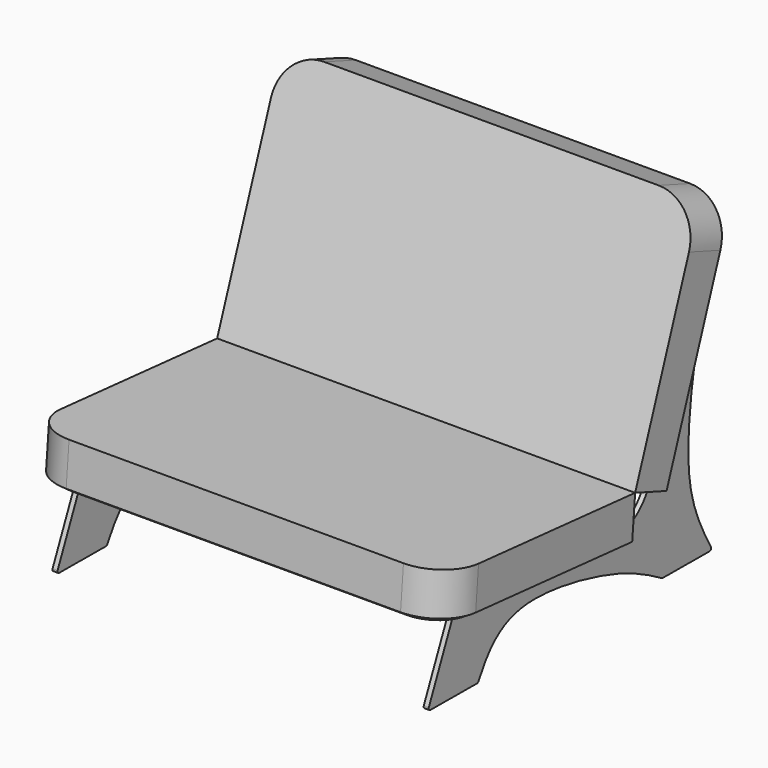
from build123d import *

# Parameters (mm, degrees)
F1_DEPTH      = 500
F1_DEPTH_BACK = 500
F2_R          = 100
F2_2_R        = 100
F4_DEPTH      = 12
F6_DEPTH      = 12
F8_START      = 438
F8_DEPTH      = 12
F10_DEPTH     = 12
F12_DEPTH     = 12
F13_R         = 5
F14_R         = 2
F15_R         = 5
F15_2_R       = 5


with BuildPart() as f1:
    # F0 (on Right) → F1 (new body, two sides)
    with BuildSketch(Plane.YZ) as f1_sk:
        Polygon((-567.8027826631, 50), (0, 0), (8.7719298246, 99.6145232742), (-559.0308528386, 149.6145232742), align=None)
    extrude(amount=F1_DEPTH)
    extrude(f1_sk.sketch, amount=-F1_DEPTH_BACK)

    # F2
    f2_edges = [f1.edges().sort_by_distance(p)[0] for p in [
        (-500, -563.416818, 99.807262),
        (500, -563.416818, 99.807262),
    ]]
    fillet(f2_edges, radius=F2_R)


with BuildPart() as f1b:
    # F0 (on Right) → F1, piece 2 (new body, two sides)
    with BuildSketch(Plane.YZ) as f1_2_sk:
        Polygon((204.0263951544, 635.1289430322), (8.7719298246, 99.6145232742), (102.7218280277, 65.3593539181), (297.9762933576, 600.8737736761), align=None)
    extrude(amount=F1_DEPTH)
    extrude(f1_2_sk.sketch, amount=-F1_DEPTH_BACK)

    # F2#2
    f2_2_edges = [f1b.edges().sort_by_distance(p)[0] for p in [
        (500, 251.001344, 618.001358),
        (-500, 251.001344, 618.001358),
    ]]
    fillet(f2_2_edges, radius=F2_2_R)


with BuildPart() as f4:
    # F3 (on face) → F4 (new body)
    with BuildSketch(Plane(origin=(0, 0, 0), x_dir=(1, 0, 0), z_dir=(0, -0.0877192982, -0.9961452327))):
        with BuildLine():
            Line((-480, 20), (480, 20))
            Line((480, 20), (480, 470))
            ThreePointArc((480, 470), (456.5685424949, 526.5685424949), (400, 550))
            Line((400, 550), (-400, 550))
            ThreePointArc((-400, 550), (-456.5685424949, 526.5685424949), (-480, 470))
            Line((-480, 470), (-480, 20))
        make_face()
    extrude(amount=F4_DEPTH)

    # F9 (on face) → F10 (cut, through all)
    with BuildSketch(Plane(origin=(0, 0, 0), x_dir=(1, 0, 0), z_dir=(0, 0.0877192982, 0.9961452327))):
        with BuildLine():
            Line((438, -51), (438, -79))
            ThreePointArc((438, -79), (437.2928932188, -80.7071067812), (439, -80))
            Line((439, -80), (449, -80))
            ThreePointArc((449, -80), (450.7071067812, -80.7071067812), (450, -79))
            Line((450, -79), (450, -51))
            ThreePointArc((450, -51), (450.7071067812, -49.2928932188), (449, -50))
            Line((449, -50), (439, -50))
            ThreePointArc((439, -50), (437.2928932188, -49.2928932188), (438, -51))
        make_face()
        with BuildLine():
            Line((438, -411), (438, -439))
            ThreePointArc((438, -439), (437.2928932188, -440.7071067812), (439, -440))
            Line((439, -440), (449, -440))
            ThreePointArc((449, -440), (450.7071067812, -440.7071067812), (450, -439))
            Line((450, -439), (450, -411))
            ThreePointArc((450, -411), (450.7071067812, -409.2928932188), (449, -410))
            Line((449, -410), (439, -410))
            ThreePointArc((439, -410), (437.2928932188, -409.2928932188), (438, -411))
        make_face()
        with BuildLine():
            ThreePointArc((-449, -410), (-450.7071067812, -409.2928932188), (-450, -411))
            Line((-450, -411), (-450, -439))
            ThreePointArc((-450, -439), (-450.7071067812, -440.7071067812), (-449, -440))
            Line((-449, -440), (-439, -440))
            ThreePointArc((-439, -440), (-437.2928932188, -440.7071067812), (-438, -439))
            Line((-438, -439), (-438, -411))
            ThreePointArc((-438, -411), (-437.2928932188, -409.2928932188), (-439, -410))
            Line((-439, -410), (-449, -410))
        make_face()
        with BuildLine():
            ThreePointArc((-450, -79), (-450.7071067812, -80.7071067812), (-449, -80))
            Line((-449, -80), (-439, -80))
            ThreePointArc((-439, -80), (-437.2928932188, -80.7071067812), (-438, -79))
            Line((-438, -79), (-438, -51))
            ThreePointArc((-438, -51), (-437.2928932188, -49.2928932188), (-439, -50))
            Line((-439, -50), (-449, -50))
            ThreePointArc((-449, -50), (-450.7071067812, -49.2928932188), (-450, -51))
            Line((-450, -51), (-450, -79))
        make_face()
    extrude(amount=-F10_DEPTH, mode=Mode.SUBTRACT)

    # F15
    f15_edges = [f4.edges().sort_by_distance(p)[0] for p in [
        (-480, -20.44922, -4.222485),
        (480, -20.44922, -4.222485),
    ]]
    fillet(f15_edges, radius=F15_R)


with BuildPart() as f6:
    # F5 (on face) → F6 (new body)
    with BuildSketch(Plane(origin=(0, 69.6338752627, -25.3892791335), x_dir=(-1, 0, 0), z_dir=(0, 0.939498982, -0.3425516936))):
        with BuildLine():
            Line((400, 646.5925826289), (-400, 646.5925826289))
            ThreePointArc((-400, 646.5925826289), (-456.5685424949, 623.1611251238), (-480, 566.5925826289))
            Line((-480, 566.5925826289), (-480, 346.5925826289))
            Line((-480, 346.5925826289), (480, 346.5925826289))
            Line((480, 346.5925826289), (480, 566.5925826289))
            ThreePointArc((480, 566.5925826289), (456.5685424949, 623.1611251238), (400, 646.5925826289))
        make_face()
    extrude(amount=F6_DEPTH)

    # F11 (on face) → F12 (cut, through all)
    with BuildSketch(Plane(origin=(0, 69.6338752627, -25.3892791335), x_dir=(1, 0, 0), z_dir=(0, -0.939498982, 0.3425516936))):
        with BuildLine():
            Line((449, 406.5925826289), (439, 406.5925826289))
            ThreePointArc((439, 406.5925826289), (437.2928932188, 407.2996894101), (438, 405.5925826289))
            Line((438, 405.5925826289), (438, 377.5925826289))
            ThreePointArc((438, 377.5925826289), (437.2928932188, 375.8854758477), (439, 376.5925826289))
            Line((439, 376.5925826289), (449, 376.5925826289))
            ThreePointArc((449, 376.5925826289), (450.7071067812, 375.8854758477), (450, 377.5925826289))
            Line((450, 377.5925826289), (450, 405.5925826289))
            ThreePointArc((450, 405.5925826289), (450.7071067812, 407.2996894101), (449, 406.5925826289))
        make_face()
        with BuildLine():
            ThreePointArc((450, 575.5925826289), (450.7071067812, 577.2996894101), (449, 576.5925826289))
            Line((449, 576.5925826289), (439, 576.5925826289))
            ThreePointArc((439, 576.5925826289), (437.2928932188, 577.2996894101), (438, 575.5925826289))
            Line((438, 575.5925826289), (438, 547.5925826289))
            ThreePointArc((438, 547.5925826289), (437.2928932188, 545.8854758477), (439, 546.5925826289))
            Line((439, 546.5925826289), (449, 546.5925826289))
            ThreePointArc((449, 546.5925826289), (450.7071067812, 545.8854758477), (450, 547.5925826289))
            Line((450, 547.5925826289), (450, 575.5925826289))
        make_face()
        with BuildLine():
            ThreePointArc((-439, 546.5925826289), (-437.2928932188, 545.8854758477), (-438, 547.5925826289))
            Line((-438, 547.5925826289), (-438, 575.5925826289))
            ThreePointArc((-438, 575.5925826289), (-437.2928932188, 577.2996894101), (-439, 576.5925826289))
            Line((-439, 576.5925826289), (-449, 576.5925826289))
            ThreePointArc((-449, 576.5925826289), (-450.7071067812, 577.2996894101), (-450, 575.5925826289))
            Line((-450, 575.5925826289), (-450, 547.5925826289))
            ThreePointArc((-450, 547.5925826289), (-450.7071067812, 545.8854758477), (-449, 546.5925826289))
            Line((-449, 546.5925826289), (-439, 546.5925826289))
        make_face()
        with BuildLine():
            ThreePointArc((-439, 376.5925826289), (-437.2928932188, 375.8854758477), (-438, 377.5925826289))
            Line((-438, 377.5925826289), (-438, 405.5925826289))
            ThreePointArc((-438, 405.5925826289), (-437.2928932188, 407.2996894101), (-439, 406.5925826289))
            Line((-439, 406.5925826289), (-449, 406.5925826289))
            ThreePointArc((-449, 406.5925826289), (-450.7071067812, 407.2996894101), (-450, 405.5925826289))
            Line((-450, 405.5925826289), (-450, 377.5925826289))
            ThreePointArc((-450, 377.5925826289), (-450.7071067812, 375.8854758477), (-449, 376.5925826289))
            Line((-449, 376.5925826289), (-439, 376.5925826289))
        make_face()
    extrude(amount=-F12_DEPTH, mode=Mode.SUBTRACT)

    # F15#2
    f15_2_edges = [f6.edges().sort_by_distance(p)[0] for p in [
        (480, 193.996745, 298.178789),
        (-480, 193.996745, 298.178789),
    ]]
    fillet(f15_2_edges, radius=F15_2_R)


with BuildPart() as f8:
    # F7 (on Right) → F8 (new body)
    with BuildSketch(Plane.YZ.offset(F8_START)):
        with BuildLine():
            Line((-469.2408909678, 29.2743273825), (-548.9325095872, -150.4562124101))
            Line((-548.9325095872, -150.4562124101), (-398.9355784863, -151.415722857))
            add(Edge.make_bspline(
                [(-398.9355784863, -151.415722857), (-387.0378707136, -130.6039570008), (-360.6274588017, -84.4062087134), (-259.1783968626, -20.3381873459), (26.4661471639, -82.1287647548), (115.2176264434, -133.4431085716), (152.4023161698, -154.9425581451)],
                knots=[0, 0, 0, 0, 0.1780865798, 0.3953147966, 0.7466517533, 1, 1, 1, 1], degree=3))
            Line((152.4023161698, -154.9425581451), (302.3992472708, -155.902068592))
            add(Edge.make_bspline(
                [(307.4871591689, 533.5421805603), (263.5046897437, 345.3277730096), (191.922790634, 39.0069841056), (271.656694879, -101.6642522591), (302.3992472708, -155.902068592)],
                knots=[0, 0, 0, 0, 0.6144356321, 1, 1, 1, 1], degree=3))
            Line((307.4871591689, 533.5421805603), (288.6971795283, 540.3932144315))
            Line((288.6971795283, 540.3932144315), (278.4206287215, 512.2082449705))
            Line((278.4206287215, 512.2082449705), (267.1466409371, 516.3188652933))
            Line((267.1466409371, 516.3188652933), (256.8700901303, 488.1338958323))
            Line((256.8700901303, 488.1338958323), (268.1440779146, 484.0232755096))
            Line((268.1440779146, 484.0232755096), (220.1868408161, 352.4934180252))
            Line((220.1868408161, 352.4934180252), (208.9128530317, 356.6040383479))
            Line((208.9128530317, 356.6040383479), (198.6363022249, 328.419068887))
            Line((198.6363022249, 328.419068887), (209.9102900092, 324.3084485642))
            Line((209.9102900092, 324.3084485642), (199.6337392024, 296.1234791033))
            Line((199.6337392024, 296.1234791033), (188.359751418, 300.234099426))
            Line((188.359751418, 300.234099426), (102.7218280277, 65.3593539181))
            Line((102.7218280277, 65.3593539181), (113.9958158121, 61.2487335954))
            ThreePointArc((113.9958158121, 61.2487335954), (68.8960383013, 5.12065268), (-1.0526315789, -11.9537427929))
            Line((-1.0526315789, -11.9537427929), (-20.9755362338, -10.199356828))
            Line((-20.9755362338, -10.199356828), (-50.8598932161, -7.5677778806))
            Line((-50.8598932161, -7.5677778806), (-49.8072616371, 4.3859649123))
            Line((-49.8072616371, 4.3859649123), (-79.6916186194, 7.0175438596))
            Line((-79.6916186194, 7.0175438596), (-80.7442501983, -4.9361989333))
            Line((-80.7442501983, -4.9361989333), (-409.4721770033, 24.0111694878))
            Line((-409.4721770033, 24.0111694878), (-408.4195454244, 35.9649122807))
            Line((-408.4195454244, 35.9649122807), (-438.3039024066, 38.5964912281))
            Line((-438.3039024066, 38.5964912281), (-439.3565339856, 26.6427484352))
            Line((-439.3565339856, 26.6427484352), (-469.2408909678, 29.2743273825))
        make_face()
    extrude(amount=F8_DEPTH)

    # F13
    f13_edges = [f8.edges().sort_by_distance(p)[0] for p in [
        (444, -548.93251, -150.456212),
        (444, -398.935578, -151.415723),
        (444, 152.402316, -154.942558),
        (444, 302.399247, -155.902069),
        (444, 307.487159, 533.542181),
    ]]
    fillet(f13_edges, radius=F13_R)

    # F14
    f14_edges = [f8.edges().sort_by_distance(p)[0] for p in [
        (444, -469.240891, 29.274327),
        (444, -438.303902, 38.596491),
        (444, -408.419545, 35.964912),
        (444, -79.691619, 7.017544),
        (444, -49.807262, 4.385965),
        (444, 113.995816, 61.248734),
        (444, 102.721828, 65.359354),
        (444, 188.359751, 300.234099),
        (444, 198.636302, 328.419069),
        (444, 208.912853, 356.604038),
        (444, 256.87009, 488.133896),
        (444, 267.146641, 516.318865),
        (444, 288.69718, 540.393214),
    ]]
    fillet(f14_edges, radius=F14_R)


with BuildPart() as f16_1:
    # F16: instance of F8
    add(f8.part.mirror(Plane.YZ))


solid = Compound([f1.part, f1b.part, f4.part, f6.part, f8.part, f16_1.part])
